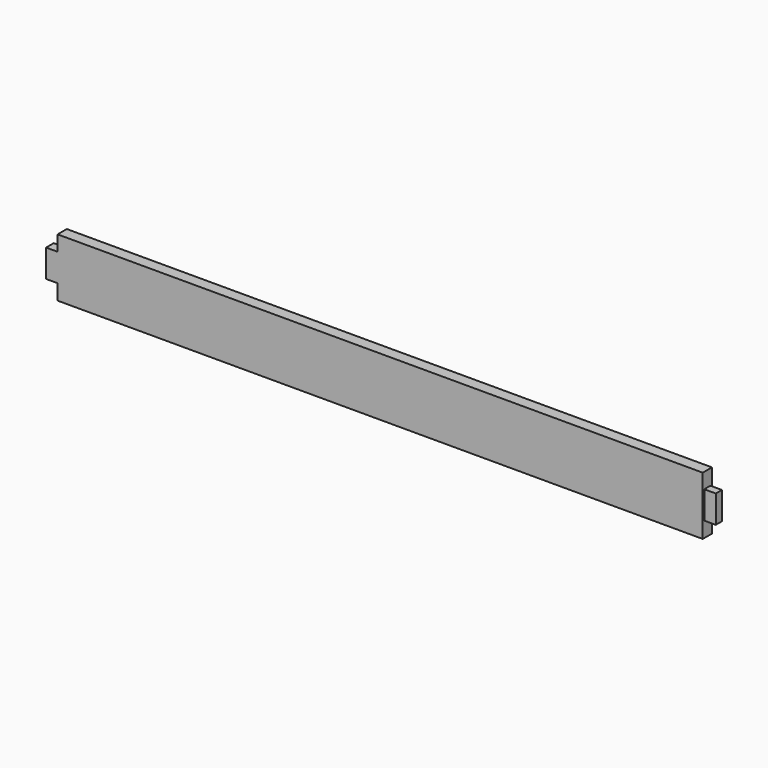
from build123d import *

# Parameters (mm, degrees)
F0_W      = 1104.9
F0_H      = 96.52
F1_DEPTH  = 19.05
F2_W      = 19.05
F2_H      = 25.4
F3_DEPTH  = 19.05
F4_W      = 19.05
F4_H      = 25.4
F5_DEPTH  = 19.05
F6_W      = 3.175
F6_H      = 45.72
F7_DEPTH  = 19.05
F8_W      = 19.05
F8_H      = 25.4
F9_DEPTH  = 19.05
F10_W     = 19.05
F10_H     = 25.4
F11_DEPTH = 19.05
F12_W     = 3.175
F12_H     = 45.72
F13_DEPTH = 19.05
F14_W     = 3.175
F14_H     = 45.72
F15_DEPTH = 19.05


# Not quite as in the source:
# - a length typed as a fraction of an inch, garbled in the dataset ("3 / 203.2 mm" for 3/8 in), is restored


with BuildPart() as f1:
    # F0 (on Front) → F1 (new body)
    with BuildSketch(Plane.XZ):
        with Locations((0, -48.26)):
            Rectangle(F0_W, F0_H)
    extrude(amount=F1_DEPTH)

    # F2 (on face) → F3 (cut)
    with BuildSketch(Plane(origin=(-552.45, 0, 0), x_dir=(0, -1, 0), z_dir=(-1, 0, 0))):
        with Locations((9.525, -12.7)):
            Rectangle(F2_W, F2_H)
    extrude(amount=-F3_DEPTH, mode=Mode.SUBTRACT)

    # F4 (on face) → F5 (cut)
    with BuildSketch(Plane(origin=(-552.45, 0, 0), x_dir=(0, -1, 0), z_dir=(-1, 0, 0))):
        with Locations((9.525, -83.82)):
            Rectangle(F4_W, F4_H)
    extrude(amount=-F5_DEPTH, mode=Mode.SUBTRACT)

    # F6 (on face) → F7 (cut)
    with BuildSketch(Plane(origin=(-552.45, 0, 0), x_dir=(0, -1, 0), z_dir=(-1, 0, 0))):
        with Locations((1.5875, -48.26)):
            Rectangle(F6_W, F6_H)
    extrude(amount=-F7_DEPTH, mode=Mode.SUBTRACT)

    # F8 (on face) → F9 (cut)
    with BuildSketch(Plane.YZ.offset(552.45)):
        with Locations((-9.525, -12.7)):
            Rectangle(F8_W, F8_H)
    extrude(amount=-F9_DEPTH, mode=Mode.SUBTRACT)

    # F10 (on face) → F11 (cut)
    with BuildSketch(Plane.YZ.offset(552.45)):
        with Locations((-9.525, -83.82)):
            Rectangle(F10_W, F10_H)
    extrude(amount=-F11_DEPTH, mode=Mode.SUBTRACT)

    # F12 (on face) → F13 (cut)
    with BuildSketch(Plane.YZ.offset(552.45)):
        with Locations((-17.4625, -48.26)):
            Rectangle(F12_W, F12_H)
    extrude(amount=-F13_DEPTH, mode=Mode.SUBTRACT)

    # F14 (on face) → F15 (cut)
    with BuildSketch(Plane.YZ.offset(552.45)):
        with Locations((-1.5875, -48.26)):
            Rectangle(F14_W, F14_H)
    extrude(amount=-F15_DEPTH, mode=Mode.SUBTRACT)


solid = f1.part
